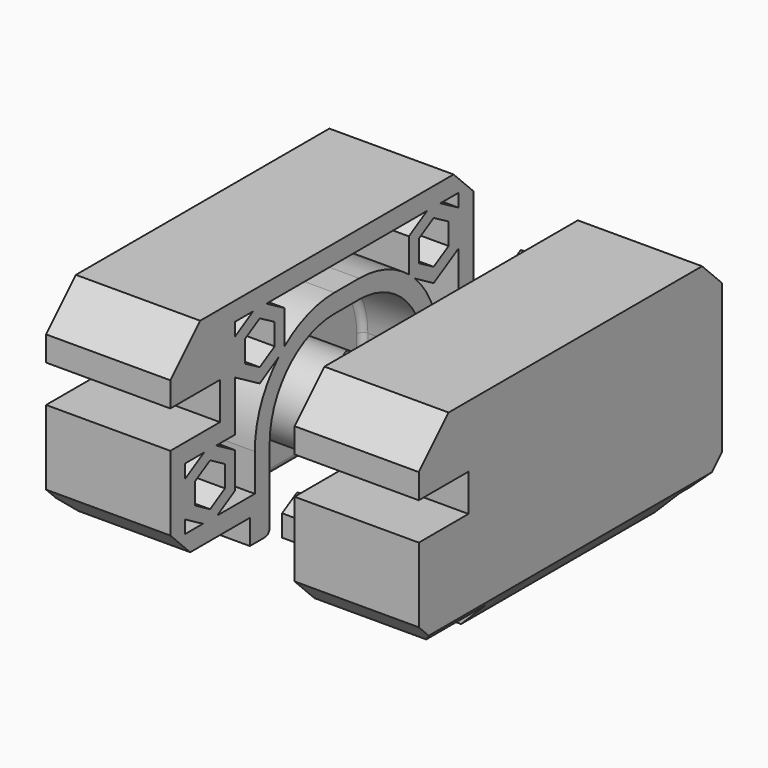
from build123d import *

# Parameters (mm, degrees)
F0_R      = 3.5
F1_DEPTH  = 10
F2_DEPTH  = 5
F4_DEPTH  = 10
F6_DEPTH  = 5
F8_DEPTH  = 5
F9_DEPTH  = 3
F10_DEPTH = 3
F11_DEPTH = 3
F13_DEPTH = 10
F14_W     = 5
F14_H     = 8.0000000403
F15_DEPTH = 10
F17_DEPTH = 3
F18_DEPTH = 3
F19_SIZE  = 2
F21_DEPTH = 10
F22_F1_R  = 0.5
F22_F2_R  = 0.5
F23_SIZE  = 3
F24_W     = 5
F24_H     = 5
F25_DEPTH = 10
F26_SIZE  = 3
F29_DEPTH = 6
F30_DEPTH = 10
F31_R     = 0.5


# Not quite as in the source:
# - ends of sketch curves that miss each other by under 0.0002 mm in the source are joined


with BuildPart() as f1:
    # F0 (on Right) → F1 (new body)
    with BuildSketch(Plane.YZ):
        with BuildLine():
            Line((4.4444442726, 0.5911923029), (4.4444442726, 6.0911924504))
            ThreePointArc((4.4444442726, 6.0911924504), (2.9799782396, 9.6267262088), (-0.5555555188, 11.0911922418))
            Line((-0.5555555188, 11.0911922418), (-3.0555555188, 11.0911922418))
            ThreePointArc((-3.0555555188, 11.0911922418), (-6.5910892772, 9.6267262088), (-8.0555553102, 6.0911924504))
            Line((-8.0555553102, 6.0911924504), (-8.0555553102, 0.5911923029))
            Line((-8.0555553102, 0.5911923029), (-8.0555554518, -0.4088076971))
            Line((-8.0555554518, -0.4088076971), (4.4444444142, -0.4088076971))
            Line((4.4444444142, -0.4088076971), (4.4444442726, 0.5911923029))
        make_face()
        with Locations((-1.8055555188, 5.3411922418)):
            Circle(F0_R, mode=Mode.SUBTRACT)
        with BuildLine():
            ThreePointArc((-0.5555555188, 11.0911922418), (2.9799782396, 9.6267262088), (4.4444442726, 6.0911924504))
            Line((4.4444442726, 6.0911924504), (4.4444442726, 0.5911923029))
            Line((4.4444442726, 0.5911923029), (4.4444444142, -0.4088076971))
            ThreePointArc((4.4444444142, -0.4088076971), (5.8586579766, 0.1769787405), (6.4444444142, 1.5911923029))
            Line((6.4444444142, 1.5911923029), (6.4444444142, 6.0911924504))
            ThreePointArc((6.4444444142, 6.0911924504), (4.3941919022, 11.0409398713), (-0.5555555188, 13.0911923834))
            Line((-0.5555555188, 13.0911923834), (-3.0555555188, 13.0911923834))
            ThreePointArc((-3.0555555188, 13.0911923834), (-8.0053029397, 11.0409398713), (-10.0555554518, 6.0911924504))
            Line((-10.0555554518, 6.0911924504), (-10.0555554518, 1.5911923029))
            ThreePointArc((-10.0555554518, 1.5911923029), (-9.4697690142, 0.1769787405), (-8.0555554518, -0.4088076971))
            Line((-8.0555554518, -0.4088076971), (-8.0555553102, 0.5911923029))
            Line((-8.0555553102, 0.5911923029), (-8.0555553102, 6.0911924504))
            ThreePointArc((-8.0555553102, 6.0911924504), (-6.5910892772, 9.6267262088), (-3.0555555188, 11.0911922418))
            Line((-3.0555555188, 11.0911922418), (-0.5555555188, 11.0911922418))
        make_face()
        with Locations((-1.8055555188, 5.3411922418)):
            Circle(F0_R)
    extrude(amount=-F1_DEPTH)

    # F0 (on Right) → F2 (cut)
    with BuildSketch(Plane.YZ):
        with BuildLine():
            Line((4.4444442726, 0.5911923029), (4.4444442726, 6.0911924504))
            ThreePointArc((4.4444442726, 6.0911924504), (2.9799782396, 9.6267262088), (-0.5555555188, 11.0911922418))
            Line((-0.5555555188, 11.0911922418), (-3.0555555188, 11.0911922418))
            ThreePointArc((-3.0555555188, 11.0911922418), (-6.5910892772, 9.6267262088), (-8.0555553102, 6.0911924504))
            Line((-8.0555553102, 6.0911924504), (-8.0555553102, 0.5911923029))
            Line((-8.0555553102, 0.5911923029), (-8.0555554518, -0.4088076971))
            Line((-8.0555554518, -0.4088076971), (4.4444444142, -0.4088076971))
            Line((4.4444444142, -0.4088076971), (4.4444442726, 0.5911923029))
        make_face()
        with Locations((-1.8055555188, 5.3411922418)):
            Circle(F0_R, mode=Mode.SUBTRACT)
    extrude(amount=-F2_DEPTH, mode=Mode.SUBTRACT)

    # F3 (on face) → F4 (join)
    with BuildSketch(Plane.YZ):
        with BuildLine():
            Line((7.9444444096, 1.5911923029), (7.9444444096, 6.0911924504))
            ThreePointArc((7.9444444096, 6.0911924504), (5.4548520693, 12.1016000431), (-0.5555555234, 14.5911923834))
            Line((-0.5555555234, 14.5911923834), (-1.8055555211, 14.5911923834))
            Line((-1.8055555211, 14.5911923834), (-3.0555555188, 14.5911923834))
            ThreePointArc((-3.0555555188, 14.5911923834), (-9.0659631115, 12.1016000431), (-11.5555554518, 6.0911924504))
            Line((-11.5555554518, 6.0911924504), (-11.5555554518, 1.5911923029))
            ThreePointArc((-11.5555554518, 1.5911923029), (-10.9697690964, 0.176978997), (-9.5555556843, -0.4088075228))
            Line((-9.5555556843, -0.4088075228), (-8.0555554564, -0.4088076971))
            ThreePointArc((-8.0555554564, -0.4088076971), (-9.4697690142, 0.1769787405), (-10.0555554518, 1.5911923029))
            Line((-10.0555554518, 1.5911923029), (-10.0555554518, 6.0911924504))
            ThreePointArc((-10.0555554518, 6.0911924504), (-8.0053029397, 11.0409398713), (-3.0555555188, 13.0911923834))
            Line((-3.0555555188, 13.0911923834), (-0.5555555188, 13.0911923834))
            ThreePointArc((-0.5555555188, 13.0911923834), (4.3941919022, 11.0409398713), (6.4444444142, 6.0911924504))
            Line((6.4444444142, 6.0911924504), (6.4444444142, 1.5911923029))
            ThreePointArc((6.4444444142, 1.5911923029), (5.8586579766, 0.1769787405), (4.4444444142, -0.4088076971))
            Line((4.4444444142, -0.4088076971), (5.9444446421, -0.4088075228))
            ThreePointArc((5.9444446421, -0.4088075228), (7.3586580542, 0.176978997), (7.9444444096, 1.5911923029))
        make_face()
    extrude(amount=-F4_DEPTH)

    # F5 (on face) → F6 (cut)
    with BuildSketch(Plane.YZ):
        with BuildLine():
            ThreePointArc((5.9444442726, 6.0911924504), (4.0406384114, 10.6873863806), (-0.5555555188, 12.5911922418))
            Line((-0.5555555188, 12.5911922418), (-3.0555555188, 12.5911922418))
            ThreePointArc((-3.0555555188, 12.5911922418), (-7.651749449, 10.6873863806), (-9.5555553102, 6.0911924504))
            Line((-9.5555553102, 6.0911924504), (-9.5555553102, 1.0911924772))
            Line((-9.5555553102, 1.0911924772), (-9.5555556843, -0.4088075228))
            Line((-9.5555556843, -0.4088075228), (-8.0555554564, -0.4088076971))
            Line((-8.0555554564, -0.4088076971), (-8.0555553102, 0.5911923029))
            Line((-8.0555553102, 0.5911923029), (-8.0555553102, 6.0911924504))
            ThreePointArc((-8.0555553102, 6.0911924504), (-6.5910892772, 9.6267262088), (-3.0555555188, 11.0911922418))
            Line((-3.0555555188, 11.0911922418), (-0.5555555188, 11.0911922418))
            ThreePointArc((-0.5555555188, 11.0911922418), (2.9799782396, 9.6267262088), (4.4444442726, 6.0911924504))
            Line((4.4444442726, 6.0911924504), (4.4444442726, 0.5911923029))
            Line((4.4444442726, 0.5911923029), (4.4444444142, -0.4088076971))
            Line((4.4444444142, -0.4088076971), (5.9444446421, -0.4088075228))
            Line((5.9444446421, -0.4088075228), (5.9444444678, 1.0911924772))
            Line((5.9444444678, 1.0911924772), (5.9444442726, 6.0911924504))
        make_face()
    extrude(amount=-F6_DEPTH, mode=Mode.SUBTRACT)

    # F7 (on face) → F8 (cut)
    with BuildSketch(Plane.YZ):
        Polygon((-3.2489311918, 2.8411922418), (-0.3621798458, 2.8411922418), (1.0811958272, 5.3411922418), (-0.3621798458, 7.8411922418), (-3.2489311918, 7.8411922418), (-4.6923068647, 5.3411922418), align=None)
    extrude(amount=-F8_DEPTH, mode=Mode.SUBTRACT)

    # F9 (add): a face of the model
    f9_faces = [f1.faces().sort_by_distance(p)[0] for p in [
        (-5, -11.5555554518, 3.8411923766),
    ]]
    extrude(f9_faces, amount=F9_DEPTH)

    # F10 (add): a face of the model
    f10_faces = [f1.faces().sort_by_distance(p)[0] for p in [
        (-5, 7.9444444096, 3.8411923766),
    ]]
    extrude(f10_faces, amount=F10_DEPTH)

    # F11 (add): a face of the model
    f11_faces = [f1.faces().sort_by_distance(p)[0] for p in [
        (-5, -1.8055555211, 14.5911923834),
    ]]
    extrude(f11_faces, amount=F11_DEPTH)

    # F12 (on face) → F13 (join)
    with BuildSketch(Plane(origin=(-10, 0, 0), x_dir=(0, -1, 0), z_dir=(-1, 0, 0))):
        with BuildLine():
            Line((0.5555555234, 14.5911923834), (0.5555555234, 17.5911923834))
            Line((0.5555555234, 17.5911923834), (-10.9444444096, 17.5911923834))
            Line((-10.9444444096, 17.5911923834), (-10.9444444096, 6.0911924504))
            Line((-10.9444444096, 6.0911924504), (-7.9444444096, 6.0911924504))
            ThreePointArc((-7.9444444096, 6.0911924504), (-5.4548520693, 12.1016000431), (0.5555555234, 14.5911923834))
        make_face()
        with BuildLine():
            Line((14.5555554518, 17.5911923834), (3.0555555188, 17.5911923834))
            Line((3.0555555188, 17.5911923834), (3.0555555188, 14.5911923834))
            ThreePointArc((3.0555555188, 14.5911923834), (9.0659631115, 12.1016000431), (11.5555554518, 6.0911924504))
            Line((11.5555554518, 6.0911924504), (14.5555554518, 6.0911924504))
            Line((14.5555554518, 6.0911924504), (14.5555554518, 17.5911923834))
        make_face()
    extrude(amount=-F13_DEPTH)

    # F14 (on face) → F15 (join)
    with BuildSketch(Plane(origin=(-10, 0, 0), x_dir=(0, -1, 0), z_dir=(-1, 0, 0))):
        with Locations((17.0555554518, 5.591192323)):
            Rectangle(F14_W, F14_H)
    extrude(amount=-F15_DEPTH)

    # F16 (on face) → F17 (cut)
    with BuildSketch(Plane.YZ):
        Polygon((-17.0555554518, 6.4266060448), (-17.0555554518, 4.6945552372), (-15.5555554518, 3.8285298335), (-14.0555554518, 4.6945552372), (-14.0555554518, 6.4266060448), (-15.5555554518, 7.2926314486), align=None)
        Polygon((-18.0555554518, 7.003956314), (-16.1724074096, 8.0911923431), (-18.0555554518, 8.0911923431), align=None)
        Polygon((-18.0555554518, 3.0911923029), (-16.2784493865, 3.0911923029), (-18.0555554518, 4.1172049681), align=None)
        with BuildLine():
            Line((-10.5555554518, 10.7044410375), (-13.0555554518, 12.1478167104))
            Line((-13.0555554518, 12.1478167104), (-13.0555554518, 8.0911923431))
            Line((-13.0555554518, 8.0911923431), (-14.9387034941, 8.0911923431))
            Line((-14.9387034941, 8.0911923431), (-13.0555554518, 7.003956314))
            Line((-13.0555554518, 7.003956314), (-13.0555554518, 4.1172049681))
            Line((-13.0555554518, 4.1172049681), (-14.8326615172, 3.0911923029))
            Line((-14.8326615172, 3.0911923029), (-11.0555553102, 3.0911923029))
            Line((-11.0555553102, 3.0911923029), (-11.0555553102, 6.0911924504))
            ThreePointArc((-11.0555553102, 6.0911924504), (-10.4331557511, 9.1848975873), (-8.6628023792, 11.7972225335))
            Line((-8.6628023792, 11.7972225335), (-10.5555554518, 10.7044410375))
        make_face()
        Polygon((-12.0555554518, 14.4572177872), (-12.0555554518, 12.7251669796), (-10.5555554518, 11.8591415758), (-9.0555554518, 12.7251669796), (-9.0555554518, 14.4572177872), (-10.5555554518, 15.323243191), align=None)
        Polygon((-13.0555554518, 15.0345680564), (-11.2254284329, 16.0911923834), (-13.0555554518, 16.0911923834), align=None)
        with BuildLine():
            Line((4.4444444096, 15.0345680564), (6.2745714286, 16.0911923834))
            Line((6.2745714286, 16.0911923834), (-9.8856824707, 16.0911923834))
            Line((-9.8856824707, 16.0911923834), (-8.0555554518, 15.0345680564))
            Line((-8.0555554518, 15.0345680564), (-8.0555554518, 12.3361902352))
            ThreePointArc((-8.0555554518, 12.3361902352), (-5.7050852588, 13.6397014965), (-3.0555555188, 14.0911922418))
            Line((-3.0555555188, 14.0911922418), (-0.5555555188, 14.0911922418))
            ThreePointArc((-0.5555555188, 14.0911922418), (2.0939742185, 13.6397014974), (4.4444444096, 12.3361902388))
            Line((4.4444444096, 12.3361902388), (4.4444444096, 15.0345680564))
        make_face()
        with BuildLine():
            Line((7.4444442353, 3.0911923029), (9.4444444096, 3.0911923029))
            Line((9.4444444096, 3.0911923029), (9.4444444096, 12.1478167104))
            Line((9.4444444096, 12.1478167104), (6.9444444096, 10.7044410375))
            Line((6.9444444096, 10.7044410375), (5.0516913481, 11.797222527))
            ThreePointArc((5.0516913481, 11.797222527), (6.8220445355, 9.1848980119), (7.4444442726, 6.0911933803))
            Line((7.4444442726, 6.0911933803), (7.4444442353, 3.0911923029))
        make_face()
        Polygon((7.6143173907, 16.0911923834), (9.4444444096, 15.0345680564), (9.4444444096, 16.0911923834), align=None)
        Polygon((5.4444444096, 14.4572177872), (5.4444444096, 12.7251669796), (6.9444444096, 11.8591415758), (8.4444444096, 12.7251669796), (8.4444444096, 14.4572177872), (6.9444444096, 15.323243191), align=None)
    extrude(amount=-F17_DEPTH, mode=Mode.SUBTRACT)

    # F18 (cut): faces of the model
    f18_faces = [f1.faces().sort_by_distance(p)[0] for p in [
        (-3, -12.0149626212, 7.5117297722),
        (-3, -1.8055555223, 14.8702719643),
        (-3, -12.4455131122, 15.7389842744),
        (-3, -17.4631867634, 3.4331965246),
        (-3, -17.4278394377, 7.7287803334),
        (-3, 8.2414950188, 7.6892970386),
        (-3, 8.83440207, 15.7389842744),
    ]]
    extrude(f18_faces, amount=-F18_DEPTH, mode=Mode.SUBTRACT)

    # F19
    f19_edges = [f1.edges().sort_by_distance(p)[0] for p in [
        (-5, 10.944444, 17.591192),
        (-5, 10.944444, 1.591192),
        (-5, -19.555555, 1.591192),
    ]]
    chamfer(f19_edges, length=F19_SIZE)

    # F20 (on face) → F21 (join)
    with BuildSketch(Plane(origin=(-10, 0, 0), x_dir=(0, -1, 0), z_dir=(-1, 0, 0))):
        with BuildLine():
            Line((-7.9444444142, -0.4088075228), (-5.9444446467, -0.4088075228))
            ThreePointArc((-5.9444446421, -0.4088075228), (-7.3586579926, 0.1769789354), (-7.9444444096, 1.5911923029))
            Line((-7.9444444142, 1.5911923029), (-7.9444444142, -0.4088075228))
        make_face()
        with BuildLine():
            Line((11.5555554518, -0.4088075228), (11.5555554518, 1.5911923029))
            ThreePointArc((11.5555554518, 1.5911923029), (10.9697690347, 0.1769789354), (9.5555556843, -0.4088075228))
            Line((9.5555556843, -0.4088075228), (11.5555554518, -0.4088075228))
        make_face()
    extrude(amount=-F21_DEPTH)

    # F22: fillet of radius 0.5 on 7 edges, made by hand

    # F22_f1
    f22_f1_edges = [f1.edges().sort_by_distance(p)[0] for p in [
        (-5, -9.5555554972, 0.3411924772),
        (-5, -9.5555553102, 3.5911924638),
        (-5, -7.651749449, 10.6873863806),
        (-5, -1.8055555188, 12.5911922418),
        (-5, 4.0406384114, 10.6873863806),
        (-5, 5.9444443702, 3.5911924638),
        (-5, 5.9444445549, 0.3411924772),
    ]]
    fillet(f22_f1_edges, radius=F22_F1_R)

    # F22_f2
    f22_f2_edges = [f1.edges().sort_by_distance(p)[0] for p in [
        (-5, -1.8055555188, -0.4088076971),
        (-2.25, 5.9444446421, -0.4088075228),
        (-2.25, -9.5555556843, -0.4088075228),
        (-5, -8.5555555704, -0.408807639),
        (-5, 4.9444445282, -0.408807639),
        (-4.8535533906, 5.7979980327, -0.4088075398),
        (-4.8535533906, -9.4091090749, -0.4088074927),
    ]]
    fillet(f22_f2_edges, radius=F22_F2_R)

    # F23
    f23_edges = [f1.edges().sort_by_distance(p)[0] for p in [
        (-10, -1.805556, -0.408808),
    ]]
    chamfer(f23_edges, length=F23_SIZE)

    # F24 (on face) → F25 (join)
    with BuildSketch(Plane(origin=(-10, 0, 0), x_dir=(0, -1, 0), z_dir=(-1, 0, 0))):
        with Locations((17.0555554518, 15.0911923834)):
            Rectangle(F24_W, F24_H)
    extrude(amount=-F25_DEPTH)

    # F26
    f26_edges = [f1.edges().sort_by_distance(p)[0] for p in [
        (-5, -19.555555, 17.591192),
    ]]
    chamfer(f26_edges, length=F26_SIZE)


with BuildPart() as f28_1:
    # F28: instance of F1
    add(f1.part.mirror(Plane.YZ.offset(5)))

    # F29 (add): faces of the model
    f29_faces = [f28_1.faces().sort_by_distance(p)[0] for p in [
        (13, -10.5555554518, 13.5911923834),
        (13, -15.5555554518, 5.560580641),
        (13, 6.9444444096, 13.5911923834),
    ]]
    extrude(f29_faces, amount=F29_DEPTH)

    # F30 (add): a face of the model
    f30_faces = [f28_1.faces().sort_by_distance(p)[0] for p in [
        (15, -1.8055555188, 5.3411922418),
    ]]
    extrude(f30_faces, amount=F30_DEPTH)

    # F31
    f31_edges = [f28_1.edges().sort_by_distance(p)[0] for p in [
        (5, -3.970619, 4.091192),
        (5, -1.805556, 2.841192),
        (5, 0.359508, 4.091192),
        (5, 0.359508, 6.591192),
        (5, -1.805556, 7.841192),
        (5, -3.970619, 6.591192),
    ]]
    fillet(f31_edges, radius=F31_R)


solid = Compound([f1.part, f28_1.part])
